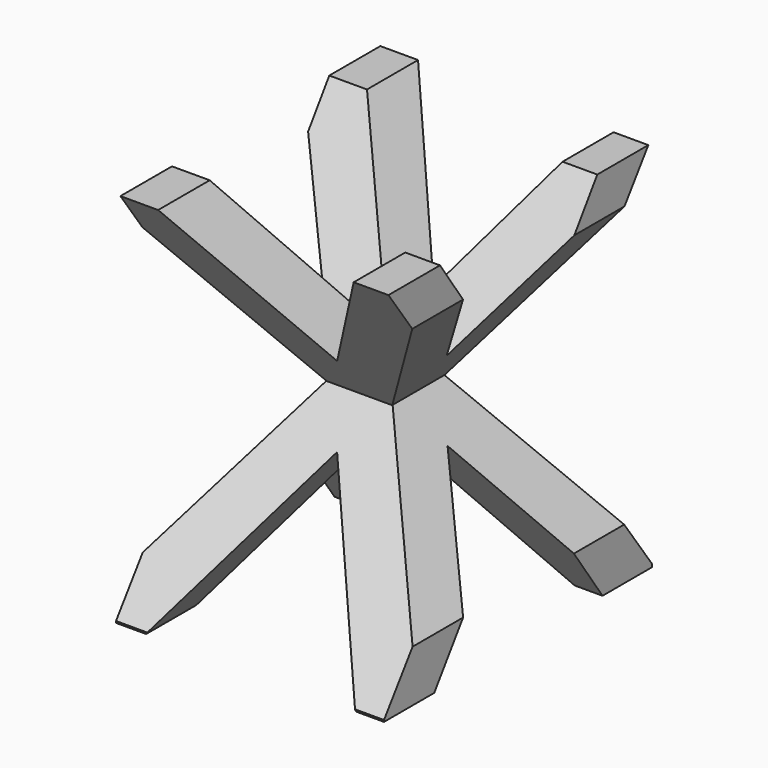
from build123d import *

# Parameters (mm, degrees)
F0_TEXT_SIZE = 133.978021978
F1_DEPTH     = 63.5
F3_START     = -25.4
F2_TEXT_SIZE = 132.2916666667
F3_DEPTH     = 50.8


# Not quite as in the source:
# - Text() gives the source's letters only with a copy of the font that has no kerning and outlines rounded to 1/6400 em; it was checked with that copy


with BuildPart() as f1:
    # F0 (on Front) → F1 (new body)
    with BuildSketch(Plane.XZ):
        with Locations((-34.8148024298, -36.2179136309)):
            Text('x', F0_TEXT_SIZE, font='Open Sans', text_align=(TextAlign.LEFT, TextAlign.BOTTOM))
    extrude(amount=F1_DEPTH)

    # F2 (on Right) → F3 (intersect)
    with BuildSketch(Plane.YZ.offset(F3_START)):
        with Locations((-66.2528732675, -35.8105564894)):
            Text('x', F2_TEXT_SIZE, font='Open Sans', text_align=(TextAlign.LEFT, TextAlign.BOTTOM))
    extrude(amount=F3_DEPTH, mode=Mode.INTERSECT)


solid = f1.part
